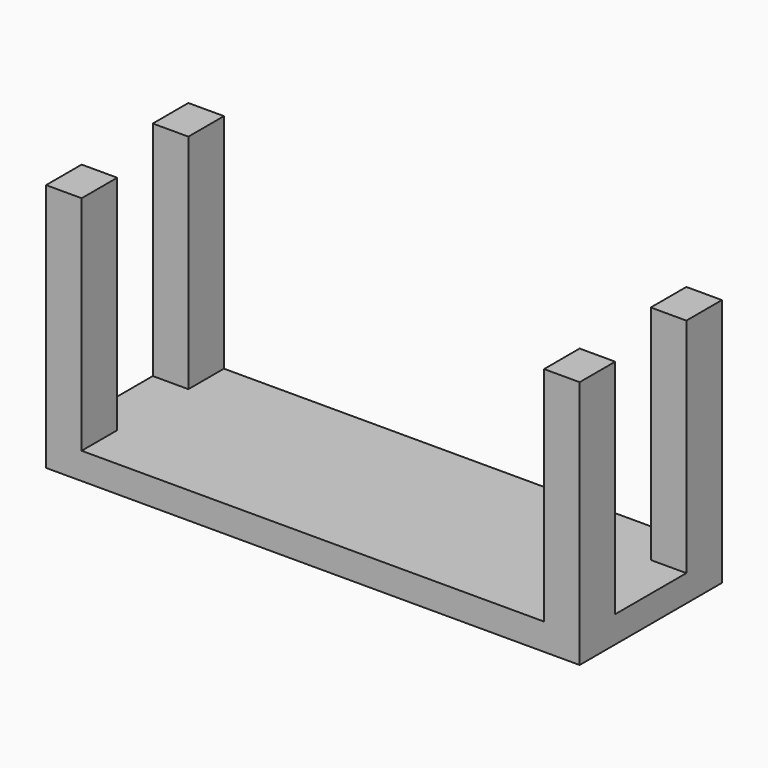
from build123d import *

# Parameters (mm, degrees)
F0_W     = 60
F0_H     = 20
F1_DEPTH = 3
F2_W     = 4
F2_H     = 20
F3_DEPTH = 25
F4_W     = 60
F4_H     = 25
F5_DEPTH = 5


# Not quite as in the source:
# - a pattern or mirror of a feature is missing from the dataset's text; its kind, count and spacing are read off the source's solid


with BuildPart() as f1:
    # F0 (on Top) → F1 (new body)
    with BuildSketch(Plane.XY):
        Rectangle(F0_W, F0_H)
    extrude(amount=F1_DEPTH)

    # F2 (on face) → F3 (join)
    with BuildSketch(Plane.XY.offset(3)):
        with Locations((-28, 0)):
            Rectangle(F2_W, F2_H)
    f3 = extrude(amount=F3_DEPTH)

    # F3_copies: F3 across plane
    add(f3.mirror(Plane(origin=(0, 0, 0), x_dir=(0, 0, 1), z_dir=(1, 0, 0))))

    # F4 (on Front) → F5 (cut, symmetric)
    with BuildSketch(Plane.XZ):
        with Locations((0, 15.5)):
            Rectangle(F4_W, F4_H)
    extrude(amount=F5_DEPTH, both=True, mode=Mode.SUBTRACT)


solid = f1.part
